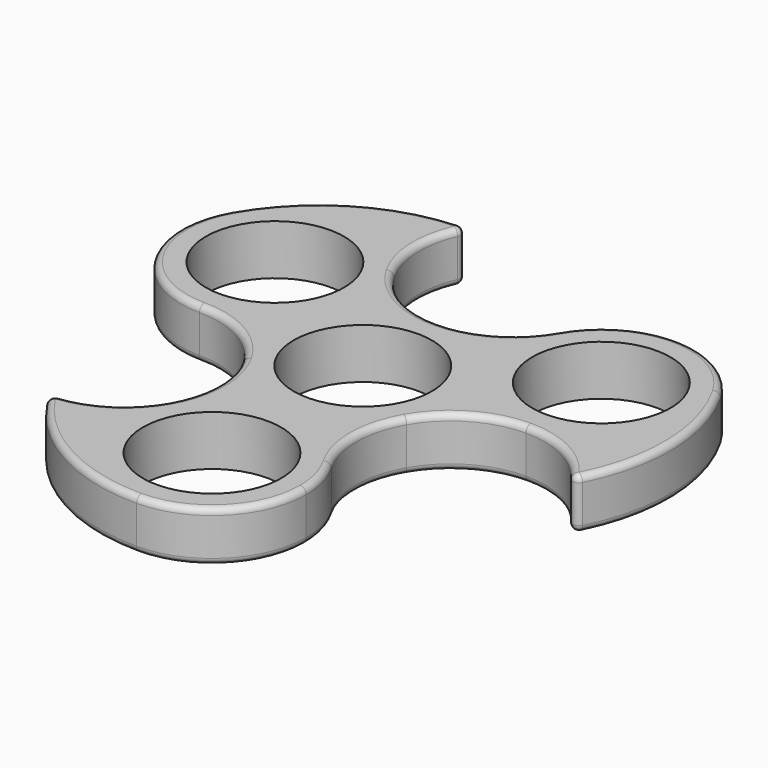
from build123d import *

# Parameters (mm, degrees)
F1_DEPTH = 8
F2_R     = 1
F3_D     = 22


# Not quite as in the source:
# - ends of sketch curves that miss each other by under 0.0002 mm in the source are joined


with BuildPart() as f1:
    # F0 (on Top) → F1 (new body)
    with BuildSketch(Plane.XY):
        with BuildLine():
            ThreePointArc((-38.9711431703, 22.5), (-25.9807619686, 30), (-12.9903809118, 22.4999997489))
            ThreePointArc((-12.9903809118, 22.4999997489), (-14.9779459784, 29.186905207), (-13.7259394882, 36.0496742725))
            ThreePointArc((-13.7259394882, 36.0496742725), (-13.8192435316, 37.0228217364), (-14.6979200558, 37.4513648462))
            ThreePointArc((-14.6979200558, 37.4513648462), (-28.723986457, 33.0431722117), (-38.9711431703, 22.5))
        make_face()
        with BuildLine():
            ThreePointArc((-12.9903809118, -22.4999997489), (-7.4999998907, -17.0096188801), (-3.74e-08, -15))
            ThreePointArc((-3.74e-08, -15), (-7.4999994973, -12.990381347), (-12.9903804576, -7.5000010378))
            ThreePointArc((-12.9903804576, -7.5000010378), (-10.9807619582, -15.0000004542), (-12.9903809118, -22.4999997489))
        make_face()
        with BuildLine():
            ThreePointArc((0, -45), (-12.9903811292, -37.4999998745), (-12.9903809118, -22.4999997489))
            ThreePointArc((-12.9903809118, -22.4999997489), (-17.7876283779, -27.5647343173), (-24.3569639741, -29.9118494238))
            ThreePointArc((-24.3569639741, -29.9118494238), (-25.1530823777, -30.4792268277), (-25.0848733353, -31.4544545742))
            ThreePointArc((-25.0848733353, -31.4544545742), (-14.2542333285, -41.3972880756), (0, -45))
        make_face()
        with BuildLine():
            ThreePointArc((12.9903809118, -22.4999997489), (10.9807619582, -15.000000145), (12.9903807668, -7.5000005022))
            ThreePointArc((12.9903807668, -7.5000005022), (7.4999999838, -12.9903810661), (-3.74e-08, -15))
            ThreePointArc((-3.74e-08, -15), (7.4999998583, -17.0096188614), (12.9903809118, -22.4999997489))
        make_face()
        with BuildLine():
            ThreePointArc((-25.9807618236, 0), (-18.4807613914, -2.0096191808), (-12.9903804576, -7.5000010378))
            ThreePointArc((-12.9903804576, -7.5000010378), (-15, -1.0077e-06), (-12.9903814652, 7.4999992925))
            ThreePointArc((-12.9903814652, 7.4999992925), (-18.4807623417, 2.0096188115), (-25.9807618236, 0))
        make_face()
        with BuildLine():
            ThreePointArc((-3.74e-08, -15), (7.4999999838, -12.9903810661), (12.9903810568, -7.5))
            ThreePointArc((12.9903810568, -7.5), (14.4888873943, -3.8822856765), (15, 0))
            ThreePointArc((15, 0), (14.488887471, 3.8822853903), (12.9903813531, 7.4999994867))
            ThreePointArc((12.9903813531, 7.4999994867), (7.5000002567, 12.9903809086), (0, 15))
            ThreePointArc((0, 15), (-7.5000003538, 12.9903808525), (-12.9903814652, 7.4999992925))
            ThreePointArc((-12.9903814652, 7.4999992925), (-15, -1.0077e-06), (-12.9903804576, -7.5000010378))
            ThreePointArc((-12.9903804576, -7.5000010378), (-7.4999994973, -12.990381347), (-3.74e-08, -15))
        make_face()
        with BuildLine():
            ThreePointArc((-12.9903814652, 7.4999992925), (-7.5000003538, 12.9903808525), (0, 15))
            ThreePointArc((0, 15), (-7.5000002032, 17.0096188812), (-12.9903809118, 22.4999997489))
            ThreePointArc((-12.9903809118, 22.4999997489), (-11.4918746817, 18.8822855365), (-10.9807621135, 15))
            ThreePointArc((-10.9807621135, 15), (-11.4918748249, 11.1177139289), (-12.9903814652, 7.4999992925))
        make_face()
        with BuildLine():
            ThreePointArc((0, 15), (7.5000002567, 12.9903809086), (12.9903813531, 7.4999994867))
            ThreePointArc((12.9903813531, 7.4999994867), (10.9807621135, 14.9999995587), (12.9903809118, 22.4999997489))
            ThreePointArc((12.9903809118, 22.4999997489), (7.5000002032, 17.0096188812), (0, 15))
        make_face()
        with BuildLine():
            ThreePointArc((-25.9807618236, 0), (-18.4807623417, 2.0096188115), (-12.9903814652, 7.4999992925))
            ThreePointArc((-12.9903814652, 7.4999992925), (-11.4918748249, 11.1177139289), (-10.9807621135, 15))
            ThreePointArc((-10.9807621135, 15), (-11.4918746817, 18.8822855365), (-12.9903809118, 22.4999997489))
            ThreePointArc((-12.9903809118, 22.4999997489), (-25.9807619686, 30), (-38.9711431703, 22.5))
            ThreePointArc((-38.9711431703, 22.5), (-38.9711430978, 7.4999998745), (-25.9807618236, 0))
        make_face()
        with BuildLine():
            ThreePointArc((40.9807621135, 15), (36.5873637288, 4.3933981797), (25.9807618236, 0))
            ThreePointArc((25.9807618236, 0), (32.7655743563, -1.6221708897), (38.0829034622, -6.1378248487))
            ThreePointArc((38.0829034622, -6.1378248487), (38.9723259093, -6.5435949088), (39.7827933911, -5.996910272))
            ThreePointArc((39.7827933911, -5.996910272), (42.9782197855, 8.3541158638), (38.9711431703, 22.5))
            ThreePointArc((38.9711431703, 22.5), (40.4696495079, 18.8822856765), (40.9807621135, 15))
        make_face()
        with BuildLine():
            ThreePointArc((12.9903813531, 7.4999994867), (18.4807622447, 2.0096188675), (25.9807618236, 0))
            ThreePointArc((25.9807618236, 0), (36.5873637288, 4.3933981797), (40.9807621135, 15))
            ThreePointArc((40.9807621135, 15), (40.4696495079, 18.8822856765), (38.9711431703, 22.5))
            ThreePointArc((38.9711431703, 22.5), (25.9807619686, 30), (12.9903809118, 22.4999997489))
            ThreePointArc((12.9903809118, 22.4999997489), (10.9807621135, 14.9999995587), (12.9903813531, 7.4999994867))
        make_face()
        with BuildLine():
            ThreePointArc((12.9903809118, -22.4999997489), (7.4999998583, -17.0096188614), (-3.74e-08, -15))
            ThreePointArc((-3.74e-08, -15), (-7.4999998907, -17.0096188801), (-12.9903809118, -22.4999997489))
            ThreePointArc((-12.9903809118, -22.4999997489), (-12.9903811292, -37.4999998745), (0, -45))
            ThreePointArc((0, -45), (10.6066017178, -40.6066017178), (15, -30))
            ThreePointArc((15, -30), (14.4888873568, -26.1177141834), (12.9903809118, -22.4999997489))
        make_face()
        with BuildLine():
            ThreePointArc((15, 0), (14.4888873943, -3.8822856765), (12.9903810568, -7.5))
            ThreePointArc((12.9903810568, -7.5), (18.4807621614, -2.0096187362), (25.9807618236, 0))
            ThreePointArc((25.9807618236, 0), (18.4807622447, 2.0096188675), (12.9903813531, 7.4999994867))
            ThreePointArc((12.9903813531, 7.4999994867), (14.488887471, 3.8822853903), (15, 0))
        make_face()
    extrude(amount=F1_DEPTH)

    # F2
    f2_edges = [f1.edges().sort_by_distance(p)[0] for p in [
        (-38.971143, 7.5, 8),
        (-13.725939, 36.049674, 4),
        (-14.69792, 37.451365, 4),
        (-13.819244, 37.022822, 0),
        (-13.819244, 37.022822, 8),
        (12.990381, -37.5, 8),
        (-38.971143, 22.5, 4),
        (-25.980762, 0, 4),
        (-38.971143, 7.5, 0),
        (-28.723986, 33.043172, 8),
        (-18.480761, -2.009619, 8),
        (-12.602933, -21.784813, 8),
        (-25.153082, -30.479227, 8),
        (-14.254233, -41.397288, 8),
        (10.980762, -15, 8),
        (25.167667, -0.022054, 8),
        (38.972326, -6.543595, 8),
        (42.97822, 8.354116, 8),
        (25.980762, 30, 8),
        (7.5, 17.009619, 8),
        (-12.564735, 21.806866, 8),
        (0, -45, 4),
        (12.990381, -22.5, 4),
        (12.990381, -37.5, 0),
        (38.971143, 22.5, 4),
        (12.990381, 22.5, 4),
        (25.980762, 30, 0),
        (-12.99038, -7.500001, 4),
        (-18.480761, -2.009619, 0),
        (0, 15, 4),
        (-12.564735, 21.806866, 0),
        (12.990381, -7.500001, 4),
        (38.082903, -6.137825, 4),
        (25.167667, -0.022054, 0),
        (-25.084873, -31.454455, 4),
        (-14.254233, -41.397288, 0),
        (-24.356964, -29.911849, 4),
        (-25.153082, -30.479227, 0),
        (39.782793, -5.99691, 4),
        (42.97822, 8.354116, 0),
        (38.972326, -6.543595, 0),
        (-28.723986, 33.043172, 0),
        (-12.602933, -21.784813, 0),
        (10.980762, -15, 0),
        (7.5, 17.009619, 0),
    ]]
    fillet(f2_edges, radius=F2_R)

    # F3 (through all)
    with Locations(Plane(origin=(0, 0, 0), x_dir=(1, 0, 0), z_dir=(0, 0, -1))):
        with Locations((-25.9807621135, -15), (25.9807621135, -15), (0, 0), (0, 30)):
            Hole(F3_D / 2)


solid = f1.part
